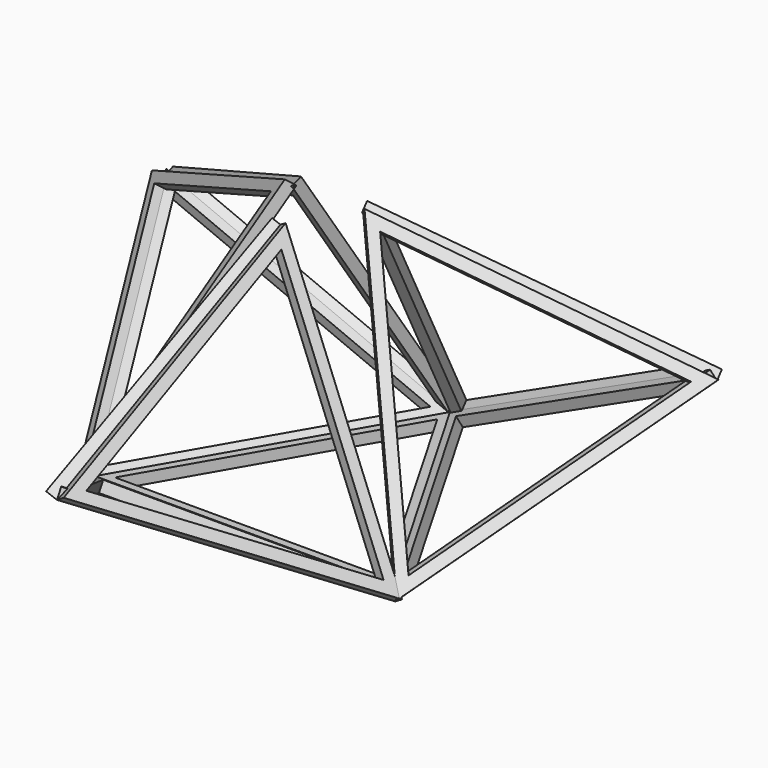
from build123d import *

# Parameters (mm, degrees)
F1_DEPTH  = 5.08
F4_DEPTH  = 5.08
F7_DEPTH  = 5.08
F10_DEPTH = 5.08
F11_ANGLE = -70
F12_ANGLE = 70
F13_ANGLE = 70
F14_ANGLE = -70
F15_ANGLE = 70
F16_ANGLE = 70


# Not quite as in the source:
# - the program builds the solid bodies; features that only make, move or delete a surface that nothing else refers to are left out


with BuildPart() as f1:
    # F0 (on Top) → F1 (new body)
    with BuildSketch(Plane.XY):
        Polygon((72.2988181024, -41.7417420935), (0, 83.4834841871), (-72.2988181024, -41.7417420935), align=None)
        Polygon((-63.5, -36.6617420935), (0, 73.3234841871), (63.5, -36.6617420935), align=None, mode=Mode.SUBTRACT)
    extrude(amount=F1_DEPTH)


with BuildPart() as f4:
    # F3 (on face) → F4 (new body)
    with BuildSketch(Plane(origin=(-9.0373522628, 5.2177177617, -18.0747045256), x_dir=(0.9013878189, 0.1200961154, -0.4160251472), z_dir=(-0.4330127019, 0.25, -0.8660254038))):
        Polygon((-134.2718128265, -89.5145418844), (10.0260421471, -80.2083371766), (-70.1822950295, 40.1041685883), align=None)
        Polygon((0.9185205239, -75.7051549814), (-125.8181818361, -83.8787878907), (-69.5284043967, 29.9652323995), align=None, mode=Mode.SUBTRACT)
    extrude(amount=-F4_DEPTH)


with BuildPart() as f7:
    # F6 (on face) → F7 (new body)
    with BuildSketch(Plane(origin=(0, -10.4354355234, -18.0747045256), x_dir=(1, 0, 0), z_dir=(0, -0.5, -0.8660254038))):
        Polygon((-72.2988181025, 36.1494090512), (72.2988181024, 36.1494090512), (0, 161.3746353318), align=None)
        Polygon((63.5, 41.2294090512), (-63.5, 41.2294090512), (0, 151.2146353318), align=None, mode=Mode.SUBTRACT)
    extrude(amount=-F7_DEPTH)


with BuildPart() as f10:
    # F9 (on face) → F10 (new body)
    with BuildSketch(Plane(origin=(9.0373522628, 5.2177177617, -18.0747045256), x_dir=(0.9013878189, -0.1200961154, 0.4160251472), z_dir=(0.4330127019, 0.25, -0.8660254038))):
        Polygon((-10.0260421471, -80.2083371766), (134.2718128265, -89.5145418844), (70.1822950295, 40.1041685883), align=None)
        Polygon((125.8181818361, -83.8787878907), (-0.9185205239, -75.7051549814), (69.5284043967, 29.9652323995), align=None, mode=Mode.SUBTRACT)
    extrude(amount=-F10_DEPTH)


with BuildPart() as f11_1:
    # F11: copy of F10
    add(f10.part.rotate(Axis((101.1835734321, 16.676621265, 31.3063065702), (-0.3995190528, -0.8080127019, -0.4330127019)), F11_ANGLE))


with BuildPart() as f12_1:
    # F12: copy of F10
    add(f10.part.rotate(Axis((65.0341643808, 79.2892344053, 31.3063065702), (-0.8995190528, 0.0580127019, -0.4330127019)), F12_ANGLE))


with BuildPart() as f13_1:
    # F13: copy of F7
    add(f7.part.rotate(Axis((-36.1494090512, -95.9658556704, 31.3063065702), (0.5, -0.75, 0.4330127019)), F13_ANGLE))


with BuildPart() as f14_1:
    # F14: copy of F7
    add(f7.part.rotate(Axis((36.1494090512, -95.9658556704, 31.3063065702), (-0.5, -0.75, 0.4330127019)), F14_ANGLE))


with BuildPart() as f15_1:
    # F15: copy of F4
    add(f4.part.rotate(Axis((-101.1835734321, 16.676621265, 31.3063065702), (0.3995190528, -0.8080127019, -0.4330127019)), F15_ANGLE))


with BuildPart() as f16_1:
    # F16: copy of F4
    add(f4.part.rotate(Axis((-65.0341643808, 79.2892344053, 31.3063065702), (-0.8995190528, -0.0580127019, 0.4330127019)), F16_ANGLE))


solid = Compound([f1.part, f4.part, f7.part, f10.part, f11_1.part, f12_1.part, f13_1.part, f14_1.part, f15_1.part, f16_1.part])
